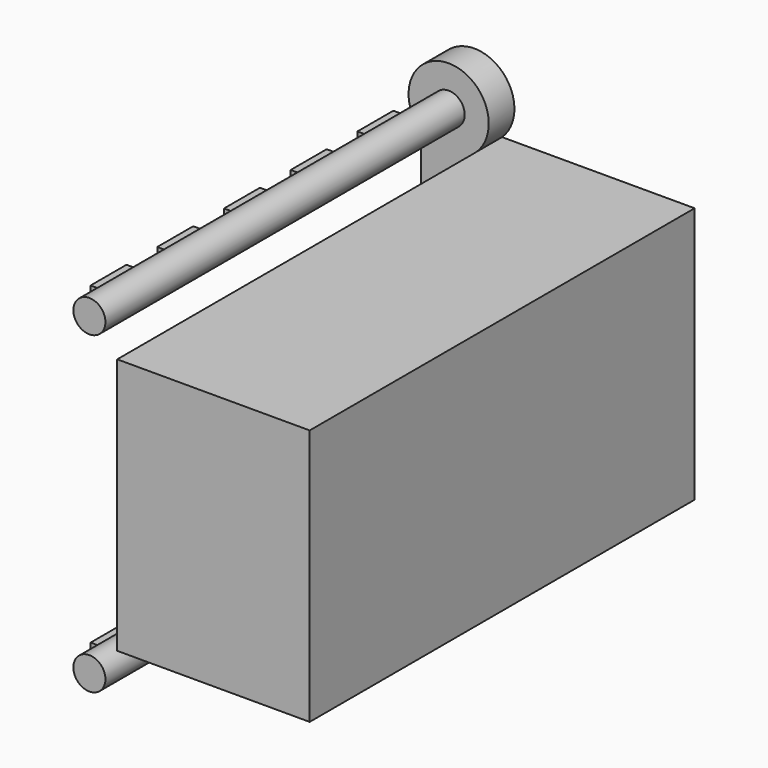
from build123d import *

# Parameters (mm, degrees)
F0_R           = 6.35
F1_DEPTH       = 177.8
F2_R           = 15.875
F2_R_2         = 6.35
F3_DEPTH       = 12.7
F6_DEPTH       = 12.7
F5_R           = 15.875
F7_DEPTH       = 12.7
F8_R           = 6.35
F9_DEPTH       = 177.8
F10_W          = 76.2
F10_H          = 101.6
F11_DEPTH      = 177.8
F11_DEPTH_BACK = 12.7
F12_W          = 165.1
F12_H          = 88.9
F13_DEPTH      = 69.85
F15_START      = 15.24
F15_DEPTH      = 17.78
F17_START      = 15.24
F17_DEPTH      = 17.78
F19_START      = 15.24
F19_DEPTH      = 17.78
F21_START      = 15.24
F21_DEPTH      = 17.78
F23_START      = 15.24
F23_DEPTH      = 17.78
F25_START      = 15.24
F25_DEPTH      = 17.78
F26_START      = 15.24
F26_DEPTH      = 17.78
F27_START      = 15.24
F27_DEPTH      = 17.78
F28_START      = 15.24
F28_DEPTH      = 17.78
F29_START      = 15.24
F29_DEPTH      = 17.78


# Not quite as in the source:
# - ends of sketch curves that miss each other by under 0.0002 mm in the source are joined


with BuildPart() as f1:
    # F0 (on Front) → F1 (new body)
    with BuildSketch(Plane.XZ):
        Circle(F0_R)
    extrude(amount=F1_DEPTH)

    # F2 (on face) → F3 (join)
    with BuildSketch(Plane(origin=(0, 0, 0), x_dir=(-1, 0, 0), z_dir=(0, 1, 0))):
        Circle(F2_R)
        Circle(F2_R_2, mode=Mode.SUBTRACT)
        Circle(F2_R_2)
    extrude(amount=F3_DEPTH)



with BuildPart() as f6:
    # F4 (on face) → F6 (new body)
    with BuildSketch(Plane(origin=(0, 12.7, 0), x_dir=(-1, 0, 0), z_dir=(0, 1, 0))):
        with BuildLine():
            ThreePointArc((-11.0168382488, 11.43), (-0.0082589267, 15.9048158213), (11.0049617512, 11.4414353057))
            Line((11.0049617512, 11.4414353057), (11.0049617512, 113.03))
            Line((11.0049617512, 113.03), (-11.0168382488, 113.03))
            Line((-11.0168382488, 113.03), (-11.0168382488, 11.43))
        make_face()
    extrude(amount=-F6_DEPTH)

    # F5 (on Front) → F7 (join)
    with BuildSketch(Plane.XZ):
        with Locations((0, 124.4932145201)):
            Circle(F5_R)
    extrude(amount=-F7_DEPTH)

    # F8 (on face) → F9 (join)
    with BuildSketch(Plane.XZ):
        with Locations((0, 124.4932145201)):
            Circle(F8_R)
    extrude(amount=F9_DEPTH)


with BuildPart() as f1_1:
    add(f1.part)

    add(f6.part)  # F11 merges F6
    # F10 (on face) → F11 (join, two sides)
    with BuildSketch(Plane.XZ) as f11_sk:
        with Locations((49.1168382488, 62.23)):
            Rectangle(F10_W, F10_H)
    extrude(amount=F11_DEPTH)
    extrude(f11_sk.sketch, amount=-F11_DEPTH_BACK)

    # F12 (on face) → F13 (cut)
    with BuildSketch(Plane(origin=(11.0168382488, 0, 0), x_dir=(0, -1, 0), z_dir=(-1, 0, 0))):
        with Locations((89.290167737, 62.6140534163)):
            Rectangle(F12_W, F12_H)
    extrude(amount=-F13_DEPTH, mode=Mode.SUBTRACT)

    # F14 (on face) → F15 (join)
    with BuildSketch(Plane.XZ.offset(F15_START)):
        with BuildLine():
            ThreePointArc((-5.9930673501, -2.0989625382), (-6.3552943125, 0), (-5.9930673501, 2.0989625382))
            ThreePointArc((-5.9930673501, 2.0989625382), (-5.9358254943, 2.2557649925), (-5.8744818664, 2.4110086688))
            Line((-5.8744818664, 2.4110086688), (-9.6825771242, 2.4110086688))
            Line((-9.6825771242, 2.4110086688), (-9.6630874508, -2.4572083608))
            Line((-9.6630874508, -2.4572083608), (-5.8553075984, -2.4572083608))
            ThreePointArc((-5.8553075984, -2.4572083608), (-5.9268948234, -2.2791265328), (-5.9930673501, -2.0989625382))
        make_face()
    extrude(amount=F15_DEPTH)


with BuildPart() as f17:
    # F16 (on face) → F17 (new body)
    with BuildSketch(Plane.XZ.offset(33.02).offset(F17_START)):
        with BuildLine():
            ThreePointArc((-5.9337336, -2.4567926286), (-6.4358893705, -0.0248806826), (-5.9533966783, 2.4110086688))
            Line((-5.9533966783, 2.4110086688), (-9.6825771242, 2.4110086688))
            Line((-9.6825771242, 2.4110086688), (-9.6630891152, -2.4567926286))
            Line((-9.6630891152, -2.4567926286), (-5.9337336, -2.4567926286))
        make_face()
    extrude(amount=F17_DEPTH)


with BuildPart() as f19:
    # F18 (on face) → F19 (new body)
    with BuildSketch(Plane.XZ.offset(66.04).offset(F19_START)):
        with BuildLine():
            ThreePointArc((-5.9739191651, -2.4566159906), (-6.4760745484, -0.0247997357), (-5.9936559097, 2.4110086688))
            Line((-5.9936559097, 2.4110086688), (-9.6825771242, 2.4110086688))
            Line((-9.6825771242, 2.4110086688), (-9.6630898224, -2.4566159906))
            Line((-9.6630898224, -2.4566159906), (-5.9739191651, -2.4566159906))
        make_face()
    extrude(amount=F19_DEPTH)


with BuildPart() as f21:
    # F20 (on face) → F21 (new body)
    with BuildSketch(Plane.XZ.offset(99.06).offset(F21_START)):
        with BuildLine():
            ThreePointArc((-5.9939809047, -2.4565356888), (-6.4961361114, -0.0247629358), (-6.0137511368, 2.4110086688))
            Line((-6.0137511368, 2.4110086688), (-9.6825771242, 2.4110086688))
            Line((-9.6825771242, 2.4110086688), (-9.6630898224, -2.4566159906))
            Line((-9.6630898224, -2.4566159906), (-5.9939809047, -2.4565356888))
        make_face()
    extrude(amount=F21_DEPTH)


with BuildPart() as f23:
    # F22 (on face) → F23 (new body)
    with BuildSketch(Plane.XZ.offset(132.08).offset(F23_START)):
        with BuildLine():
            ThreePointArc((-6.0039925358, -2.4565433546), (-6.5061477593, -0.0247664488), (-6.0237595711, 2.4110086688))
            Line((-6.0237595711, 2.4110086688), (-9.6825771242, 2.4110086688))
            Line((-9.6825771242, 2.4110086688), (-9.6630898224, -2.4566159906))
            Line((-9.6630898224, -2.4566159906), (-6.0039925358, -2.4565433546))
        make_face()
    extrude(amount=F23_DEPTH)


with BuildPart() as f25:
    # F24 (on face) → F25 (new body)
    with BuildSketch(Plane.XZ.offset(F25_START)):
        with BuildLine():
            ThreePointArc((-5.875426674, 121.9974181886), (-6.3775833502, 124.4295553562), (-5.8949163474, 126.8656352182))
            Line((-5.8949163474, 126.8656352182), (-9.7049163474, 126.8656352182))
            Line((-9.7049163474, 126.8656352182), (-9.685426674, 121.9974181886))
            Line((-9.685426674, 121.9974181886), (-5.875426674, 121.9974181886))
        make_face()
    extrude(amount=F25_DEPTH)


with BuildPart() as f26:
    # F25_face (on face) → F26 (new body)
    with BuildSketch(Plane(origin=(-7.9525870478, -33.02, 124.4316019733), x_dir=(1, 0, 0), z_dir=(0, -1, 0)).offset(F26_START)):
        with BuildLine():
            ThreePointArc((2.0771603738, -2.4341837848), (1.5750036976, -0.0020466171), (2.0576707004, 2.4340332449))
            Line((2.0576707004, 2.4340332449), (-1.7523292996, 2.4340332449))
            Line((-1.7523292996, 2.4340332449), (-1.7328396262, -2.4341837848))
            Line((-1.7328396262, -2.4341837848), (2.0771603738, -2.4341837848))
        make_face()
    extrude(amount=F26_DEPTH)


with BuildPart() as f27:
    # F26_face (on face) → F27 (new body)
    with BuildSketch(Plane(origin=(-7.9525870478, -66.04, 124.4316019733), x_dir=(1, 0, 0), z_dir=(0, -1, 0)).offset(F27_START)):
        with BuildLine():
            Line((-1.7328396262, -2.4341837848), (2.0771603738, -2.4341837848))
            ThreePointArc((2.0771603738, -2.4341837848), (1.5750036976, -0.0020466171), (2.0576707004, 2.4340332449))
            Line((2.0576707004, 2.4340332449), (-1.7523292996, 2.4340332449))
            Line((-1.7523292996, 2.4340332449), (-1.7328396262, -2.4341837848))
        make_face()
    extrude(amount=F27_DEPTH)


with BuildPart() as f28:
    # F27_face (on face) → F28 (new body)
    with BuildSketch(Plane(origin=(-7.9525870478, -99.06, 124.4316019733), x_dir=(1, 0, 0), z_dir=(0, -1, 0)).offset(F28_START)):
        with BuildLine():
            Line((2.0576707004, 2.4340332449), (-1.7523292996, 2.4340332449))
            Line((-1.7523292996, 2.4340332449), (-1.7328396262, -2.4341837848))
            Line((-1.7328396262, -2.4341837848), (2.0771603738, -2.4341837848))
            ThreePointArc((2.0771603738, -2.4341837848), (1.5750036976, -0.0020466171), (2.0576707004, 2.4340332449))
        make_face()
    extrude(amount=F28_DEPTH)


with BuildPart() as f29:
    # F28_face (on face) → F29 (new body)
    with BuildSketch(Plane(origin=(-7.9525870478, -132.08, 124.4316019733), x_dir=(1, 0, 0), z_dir=(0, -1, 0)).offset(F29_START)):
        with BuildLine():
            Line((2.0576707004, 2.4340332449), (-1.7523292996, 2.4340332449))
            Line((-1.7523292996, 2.4340332449), (-1.7328396262, -2.4341837848))
            Line((-1.7328396262, -2.4341837848), (2.0771603738, -2.4341837848))
            ThreePointArc((2.0771603738, -2.4341837848), (1.5750036976, -0.0020466171), (2.0576707004, 2.4340332449))
        make_face()
    extrude(amount=F29_DEPTH)


solid = Compound([f1_1.part, f17.part, f19.part, f21.part, f23.part, f25.part, f26.part, f27.part, f28.part, f29.part])
